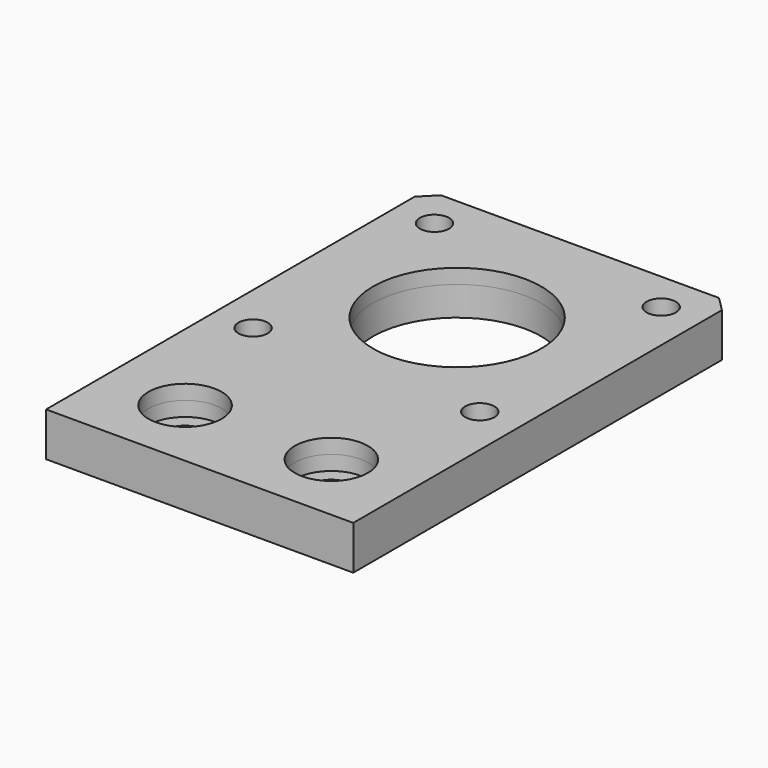
from build123d import *

# Parameters (mm, degrees)
F0_W           = 42
F0_H           = 42
F1_DEPTH       = 4
F3_D           = 4
F3_DEPTH       = 55
F3_TIP         = 1.2017212381
F4_D           = 23
F4_DEPTH       = 55
F4_TIP         = 6.9098971188
F5_DEPTH       = 23
F7_D           = 6
F7_DEPTH       = 55
F7_CBORE_D     = 10
F7_CBORE_DEPTH = 2
F7_TIP         = 1.8025818571
F8_SIZE        = 2
F9_DEPTH       = 2


with BuildPart() as f1:
    # F0 (on Top) → F1 (new body)
    with BuildSketch(Plane.XY):
        Rectangle(F0_W, F0_H)
    extrude(amount=F1_DEPTH)

    # F3
    with Locations(Plane.XY.offset(4)):
        with Locations((-15.5, 15.5), (-15.5, -15.5), (15.5, 15.5), (15.5, -15.5)):
            Hole(F3_D / 2, depth=F3_DEPTH)
            with Locations((0, 0, -(F3_DEPTH + F3_TIP / 2))):  # 118° drill point
                Cone(0, F3_D / 2, F3_TIP, mode=Mode.SUBTRACT)

    # F4
    with Locations(Plane.XY.offset(4)):
        with Locations((0, 0)):
            Hole(F4_D / 2, depth=F4_DEPTH)
            with Locations((0, 0, -(F4_DEPTH + F4_TIP / 2))):  # 118° drill point
                Cone(0, F4_D / 2, F4_TIP, mode=Mode.SUBTRACT)

    # F5 (add): a face of the model
    f5_faces = [f1.faces().sort_by_distance(p)[0] for p in [
        (0, -21, 2),
    ]]
    extrude(f5_faces, amount=F5_DEPTH)

    # F7
    with Locations(Plane.XY.offset(4)):
        with Locations((-10, -34), (10, -34)):
            CounterBoreHole(F7_D / 2, F7_CBORE_D / 2, F7_CBORE_DEPTH, depth=F7_DEPTH)
            with Locations((0, 0, -(F7_DEPTH + F7_TIP / 2))):  # 118° drill point
                Cone(0, F7_D / 2, F7_TIP, mode=Mode.SUBTRACT)

    # F8
    f8_edges = [f1.edges().sort_by_distance(p)[0] for p in [
        (21, 21, 2),
        (-21, 21, 2),
    ]]
    chamfer(f8_edges, length=F8_SIZE)

    # F9 (add): a face of the model
    f9_faces = [f1.faces().sort_by_distance(p)[0] for p in [
        (0, -12.426722897, 4),
    ]]
    extrude(f9_faces, amount=F9_DEPTH)


solid = f1.part
